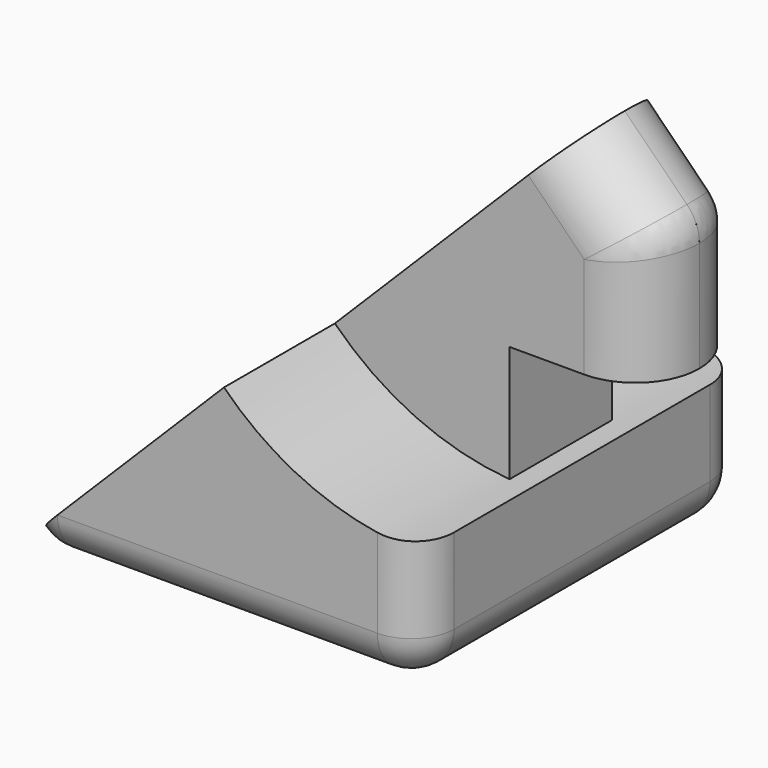
from build123d import *

# Parameters (mm, degrees)
F0_W      = 19
F0_H      = 19
F1_DEPTH  = 9.5
F3_DEPTH  = 19.001
F5_DEPTH  = 3
F6_R      = 2
F8_DEPTH  = 12.501
F9_R      = 2
F11_DEPTH = 9.5
F12_R     = 2.99999
F13_R     = 2


# Not quite as in the source:
# - a fillet or chamfer is up to 0.001 mm smaller than in the source, because OpenCascade refuses the exact size


with BuildPart() as f1:
    # F0 (on Front) → F1 (new body, symmetric)
    with BuildSketch(Plane.XZ):
        with Locations((9.5, 9.5)):
            Rectangle(F0_W, F0_H)
    extrude(amount=F1_DEPTH, both=True)

    # F2 (on face) → F3 (cut, through all)
    with BuildSketch(Plane.XZ.offset(9.5)):
        with BuildLine():
            ThreePointArc((6, 19), (9.8076118446, 9.8076118446), (19, 6))
            Line((19, 6), (19, 19))
            Line((19, 19), (6, 19))
        make_face()
    extrude(amount=-F3_DEPTH, mode=Mode.SUBTRACT)

    # F4 (on Front) → F5 (join, symmetric)
    with BuildSketch(Plane.XZ):
        Polygon((0, 18), (0, 0), (18, 0), (18, 11.5), (24.5, 11.5), (24.5, 24.5), (11.5, 24.5), (11.5, 18), align=None)
    extrude(amount=F5_DEPTH, both=True)

    # F6
    f6_edges = [f1.edges().sort_by_distance(p)[0] for p in [
        (0, 0, 0),
    ]]
    fillet(f6_edges, radius=F6_R)

    # F7 (on face) → F8 (cut, through all)
    with BuildSketch(Plane.XZ.offset(3)):
        Polygon((17.5, 24.5), (24.5, 17.5), (24.5, 24.5), align=None)
    extrude(amount=-F8_DEPTH, mode=Mode.SUBTRACT)

    # F9
    f9_edges = [f1.edges().sort_by_distance(p)[0] for p in [
        (0, -9.5, 10.5),
        (0, 9.5, 10.5),
        (0, 0, 19),
        (3, 9.5, 19),
        (3, -9.5, 19),
        (19, 9.5, 3),
        (19, 0, 0),
        (19, -9.5, 3),
    ]]
    fillet(f9_edges, radius=F9_R)

    # F10 (on Front) → F11 (cut, symmetric)
    with BuildSketch(Plane.XZ):
        Polygon((0, 25), (0, 0), (25, 25), align=None)
    extrude(amount=F11_DEPTH, both=True, mode=Mode.SUBTRACT)

    # F12 (radius 3 in the source; OpenCascade refuses exactly that, so slightly less here)
    f12_edges = [f1.edges().sort_by_distance(p)[0] for p in [
        (22.75, -3, 19.25),
        (24.5, -3, 14.5),
        (24.5, 3, 14.5),
        (22.75, 3, 19.25),
    ]]
    fillet(f12_edges, radius=F12_R)

    # F13
    f13_edges = [f1.edges().sort_by_distance(p)[0] for p in [
        (23.579023, 2.162797, 17.118519),
    ]]
    fillet(f13_edges, radius=F13_R)


solid = f1.part
